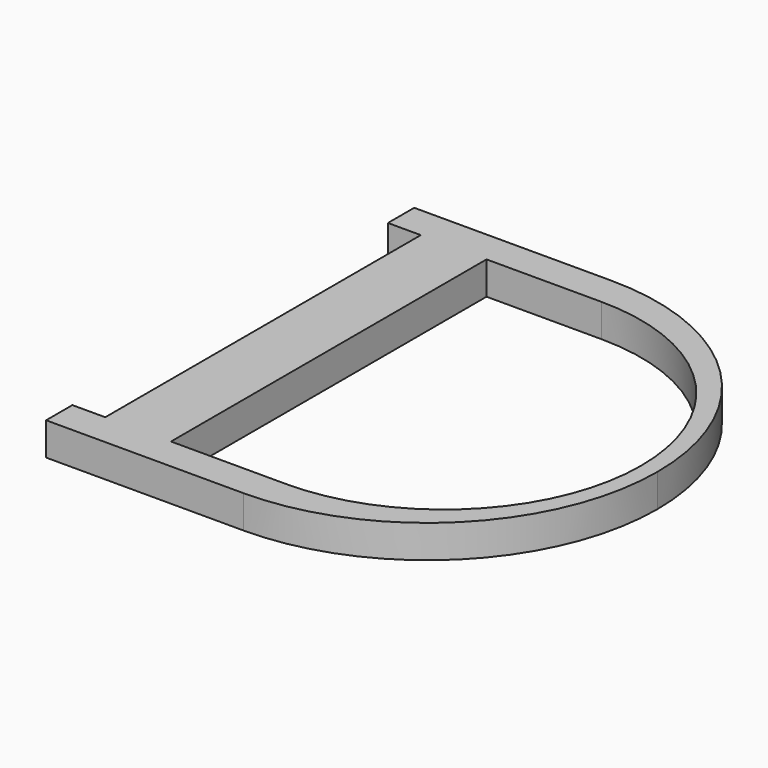
from build123d import *

# Parameters (mm, degrees)
F1_DEPTH = 6.35
F2_R     = 44.44999


# Not quite as in the source:
# - a fillet or chamfer is up to 0.001 mm smaller than in the source, because OpenCascade refuses the exact size


with BuildPart() as f1:
    # F0 (on Top) → F1 (new body)
    with BuildSketch(Plane.XY):
        Polygon((41.275, -44.45), (41.275, 44.45), (-41.275, 44.45), (-41.275, 38.1), (-34.925, 38.1), (-34.925, -38.1), (-41.275, -38.1), (-41.275, -44.45), align=None)
        with BuildLine():
            Line((0, -38.1), (-22.225, -38.1))
            Line((-22.225, -38.1), (-22.225, 38.1))
            Line((-22.225, 38.1), (0, 38.1))
            ThreePointArc((0, 38.1), (38.1, 0), (0, -38.1))
        make_face(mode=Mode.SUBTRACT)
    extrude(amount=F1_DEPTH)

    # F2 (radius 44.45 in the source; OpenCascade refuses exactly that, so slightly less here)
    f2_edges = [f1.edges().sort_by_distance(p)[0] for p in [
        (41.275, -44.45, 3.175),
        (41.275, 44.45, 3.175),
    ]]
    fillet(f2_edges, radius=F2_R)


solid = f1.part
